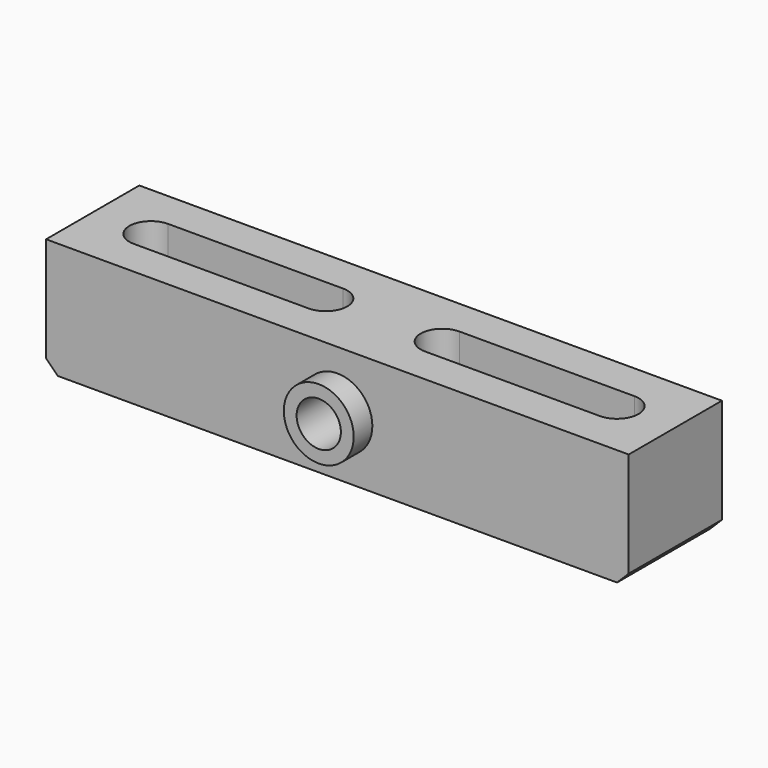
from build123d import *

# Parameters (mm, degrees)
F0_W     = 50
F0_H     = 10
F0_R     = 1.9
F1_DEPTH = 5
F2_SIZE  = 1
F4_DEPTH = 12.5
F5_R     = 3
F5_R_2   = 1.9
F6_DEPTH = 2


# Not quite as in the source:
# - a feature names something its author has since deleted; it is built from what else it names


with BuildPart() as f1:
    # F0 (on Front) → F1 (new body, symmetric)
    with BuildSketch(Plane.XZ):
        Rectangle(F0_W, F0_H)
        Circle(F0_R, mode=Mode.SUBTRACT)
    extrude(amount=F1_DEPTH, both=True)

    # F2
    f2_edges = [f1.edges().sort_by_distance(p)[0] for p in [
        (-25, 0, -5),
        (25, 0, -5),
    ]]
    chamfer(f2_edges, length=F2_SIZE)

    # F3 (on Top) → F4 (cut, symmetric)
    with BuildSketch(Plane.XY):
        with BuildLine():
            ThreePointArc((-20, 1.85), (-21.85, 0), (-20, -1.85))
            Line((-20, -1.85), (-5, -1.85))
            ThreePointArc((-5, -1.85), (-3.15, 0), (-5, 1.85))
            Line((-5, 1.85), (-20, 1.85))
        make_face()
        with BuildLine():
            Line((5, -1.85), (20, -1.85))
            ThreePointArc((20, -1.85), (21.85, 0), (20, 1.85))
            Line((20, 1.85), (5, 1.85))
            ThreePointArc((5, 1.85), (3.15, 0), (5, -1.85))
        make_face()
    extrude(amount=F4_DEPTH, both=True, mode=Mode.SUBTRACT)

    # F5 (on face) → F6 (join)
    with BuildSketch(Plane.XZ.offset(5)):
        Circle(F5_R)
        Circle(F5_R_2, mode=Mode.SUBTRACT)
    extrude(amount=F6_DEPTH)


solid = f1.part
